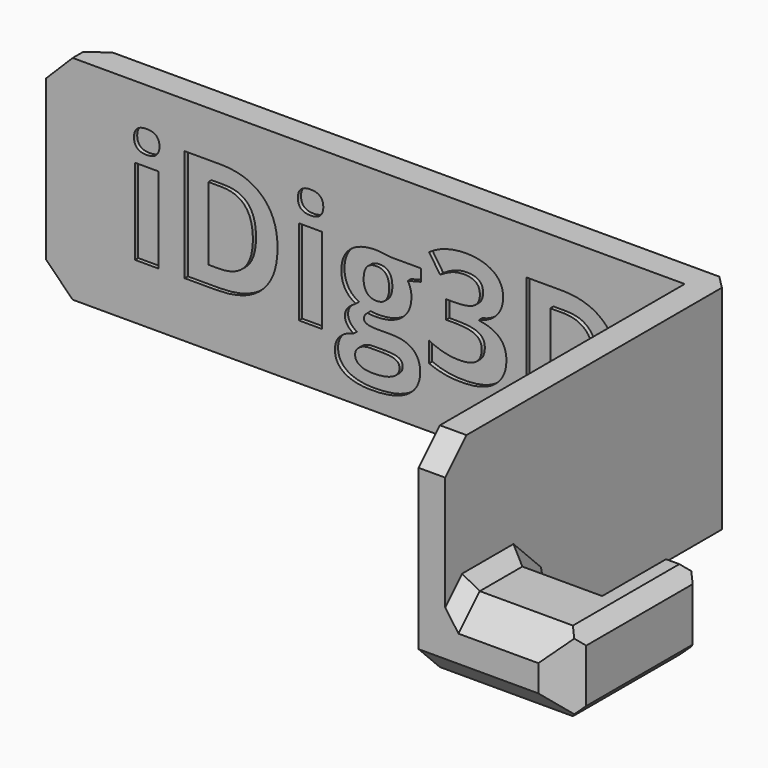
from build123d import *

# Parameters (mm, degrees)
F1_DEPTH     = 6
F2_DEPTH     = 10
F3_SIZE      = 2
F4_SIZE      = 1
F5_TEXT_SIZE = 11.7800369054
F6_DEPTH     = 0.3


# Not quite as in the source:
# - a feature names something its author has since deleted; it is built from what else it names
# - Text() gives the source's letters only with a copy of the font that has no kerning and outlines rounded to 1/6400 em; it was checked with that copy


with BuildPart() as f1:
    # F0 (on Top) → F1 (new body)
    with BuildSketch(Plane.XY):
        Polygon((0, 0), (-50, 0), (-50, -2), (-2, -2), (-2, -27), (0, -27), (0, -19), align=None)
        Polygon((6, -19), (0, -19), (0, -27), (6, -27), (9, -27), (9, -13), (6, -13), align=None)
    extrude(amount=-F1_DEPTH)

    # F0 (on Top) → F2 (join)
    with BuildSketch(Plane.XY):
        Polygon((0, 0), (-50, 0), (-50, -2), (-2, -2), (-2, -27), (0, -27), (0, -19), align=None)
    extrude(amount=F2_DEPTH)

    # F3
    f3_edges = [f1.edges().sort_by_distance(p)[0] for p in [
        (3, -19, -6),
        (3.5, -27, -6),
        (3, -19, 0),
        (4.5, -27, 0),
        (-1, -27, 10),
        (-50, -1, -6),
        (-50, -1, 10),
        (9, -27, -3),
        (7.5, -13, -6),
        (7.5, -13, 0),
        (9, -13, -3),
    ]]
    chamfer(f3_edges, length=F3_SIZE)

    # F4
    f4_edges = [f1.edges().sort_by_distance(p)[0] for p in [
        (0, -26, -1),
        (0, -23, 0),
        (0, -20, -1),
        (0, -19, -3),
        (6, -19, -3),
        (9, -20, -6),
        (9, -20, 0),
        (-50, 0, 2),
        (-49, 0, -5),
        (-49, 0, 9),
        (0, 0, 2),
        (6, -17, 0),
        (6, -17, -6),
        (0, -20, -5),
        (6, -20, -6),
        (6, -20, 0),
    ]]
    chamfer(f4_edges, length=F4_SIZE)

    # F5 (on face) → F6 (cut)
    with BuildSketch(Plane.XZ.offset(2)):
        with Locations((-44.2345734239, -1.8411766505)):
            Text('iDig3D', F5_TEXT_SIZE, font='Open Sans', font_style=FontStyle.BOLD, text_align=(TextAlign.LEFT, TextAlign.BOTTOM))
    extrude(amount=-F6_DEPTH, mode=Mode.SUBTRACT)


solid = f1.part
